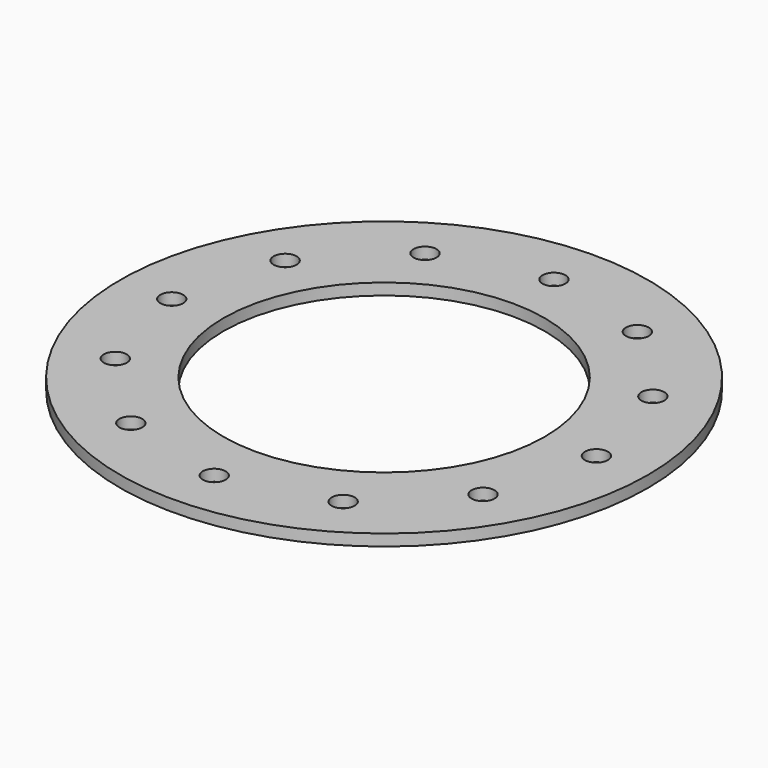
from build123d import *

# Parameters (mm, degrees)
F0_R            = 115
F0_R_2          = 70
F1_DEPTH        = 5
F2_R            = 5
F3_DEPTH        = 25
F3_COPIES_COUNT = 12


# Not quite as in the source:
# - a pattern or mirror of a feature is missing from the dataset's text; its kind, count and spacing are read off the source's solid


with BuildPart() as f1:
    # F0 (on Top) → F1 (new body)
    with BuildSketch(Plane.XY):
        Circle(F0_R)
        Circle(F0_R_2, mode=Mode.SUBTRACT)
    extrude(amount=F1_DEPTH)

    # F2 (on face) → F3 (cut)
    with BuildSketch(Plane.XY.offset(5)):
        with Locations((0, 92.5)):
            Circle(F2_R)
    f3 = extrude(amount=-F3_DEPTH, mode=Mode.SUBTRACT)

    # F3_copies: F3 ×12 about axis
    f3_copies_axis = Axis((0, 0, 0), (0, 0, 1))
    for i in range(1, F3_COPIES_COUNT):
        add(f3.rotate(f3_copies_axis, i * 360 / F3_COPIES_COUNT), mode=Mode.SUBTRACT)


solid = f1.part
